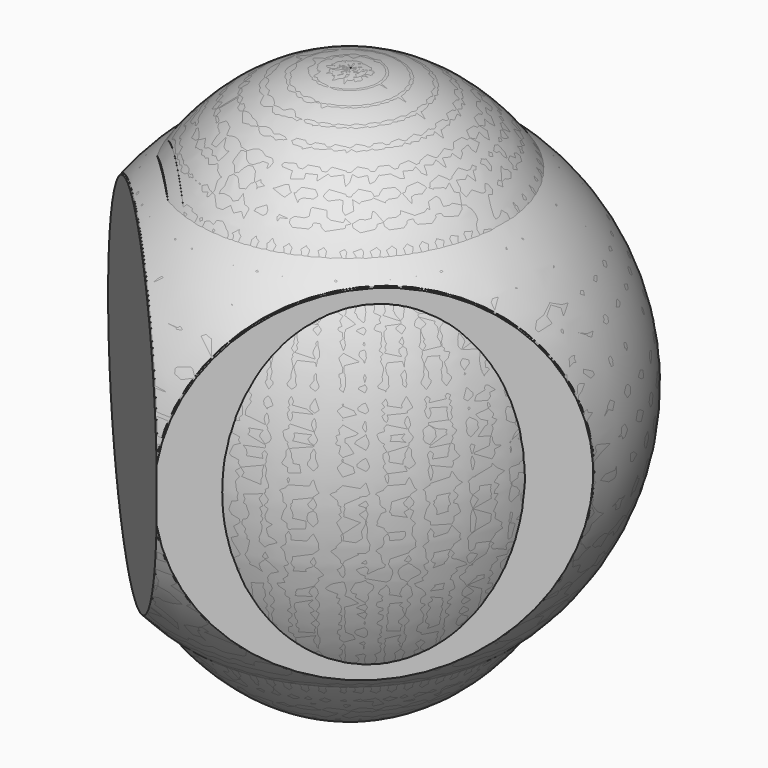
from build123d import *

# Parameters (mm, degrees)
F3_DEPTH       = 20.0010001
F3_DEPTH_BACK  = 25
F5_R           = 4
F6_DEPTH       = 8
F10_DEPTH      = 20.0010001
F10_DEPTH_BACK = 25
F13_R          = 4
F14_DEPTH      = 11.78
F18_DEPTH      = 20.0009988318
F18_DEPTH_BACK = 25
F20_R          = 4
F21_DEPTH      = 8
F25_DEPTH      = 20.0009988318
F25_DEPTH_BACK = 25
F28_R          = 4
F29_DEPTH      = 9.69
F33_R          = 1.486505693
F34_DEPTH      = 5


with BuildPart() as f1:
    # F0 (on Front) → F1 (revolve)
    with BuildSketch(Plane.XZ):
        with BuildLine():
            Line((0, 20), (0, -20))
            add(Edge.make_bspline(
                [(0, -20), (15, -20), (15, 0), (15, 20), (0, 20)],
                knots=[0, 0, 0, 1.5707963268, 1.5707963268, 3.1415926536, 3.1415926536, 3.1415926536], degree=2, weights=[1, 0.7071067812, 1, 0.7071067812, 1]))
        make_face()
    revolve(axis=Axis((0, 0, 1.515686512), (0, 0, -1)))

    # F2 (on Top) → F3 (cut, two sides)
    with BuildSketch(Plane.XY) as f3_sk:
        Polygon((1.0869333055, -18.0716644973), (1.0869333055, -15.0260711089), (-14.0562849119, 0), (1.0869333055, 14.9701479822), (1.0869333055, 17.4571201205), (-20.6206664443, 17.9764218628), (-19.673416391, -17.4401663244), align=None)
    extrude(amount=F3_DEPTH, mode=Mode.SUBTRACT)
    extrude(f3_sk.sketch, amount=-F3_DEPTH_BACK, mode=Mode.SUBTRACT)

    # F5 (on offset) → F6 (cut)
    with BuildSketch(Plane.XY.offset(-20.2)):
        Circle(F5_R)
    extrude(amount=F6_DEPTH, mode=Mode.SUBTRACT)


with BuildPart() as f8:
    # F7 (on Front) → F8 (revolve)
    with BuildSketch(Plane.XZ):
        with BuildLine():
            Line((0, 20), (0, -20))
            add(Edge.make_bspline(
                [(0, -20), (15, -20), (15, 0), (15, 20), (0, 20)],
                knots=[3.1415926536, 3.1415926536, 3.1415926536, 4.7123889804, 4.7123889804, 6.2831853072, 6.2831853072, 6.2831853072], degree=2, weights=[1, 0.7071067812, 1, 0.7071067812, 1]))
        make_face()
    revolve(axis=Axis((0, 0, 0), (0, 0, -1)))

    # F9 (on Top) → F10 (cut, two sides)
    with BuildSketch(Plane.XY) as f10_sk:
        Polygon((-19.6712000702, -17.4563237451), (2.0983788266, -17.0855390455), (-14.9871602189, 0), (3.7128583062, 18.7000185251), (-20.6184501235, 17.9602644421), align=None)
    extrude(amount=F10_DEPTH, mode=Mode.SUBTRACT)
    extrude(f10_sk.sketch, amount=-F10_DEPTH_BACK, mode=Mode.SUBTRACT)

    # F13 (on face) → F14 (cut)
    with BuildSketch(Plane(origin=(6.3216225389, 0, -23.5926165013), x_dir=(0.9659258263, 0, 0.2588190451), z_dir=(0.2588190451, 0, -0.9659258263))):
        with Locations((-1.1815404284, 0)):
            Circle(F13_R)
    extrude(amount=-F14_DEPTH, mode=Mode.SUBTRACT)


with BuildPart() as f16:
    # F15 (on Front) → F16 (revolve)
    with BuildSketch(Plane.XZ):
        with BuildLine():
            Line((0, 17.524996667), (0, -17.475003333))
            ThreePointArc((0, -17.475003333), (17.5, 0.024996667), (0, 17.524996667))
        make_face()
    revolve(axis=Axis((0, 0, 0.024996667), (0, 0, 1)))

    # F17 (on Top) → F18 (cut, two sides)
    with BuildSketch(Plane.XY) as f18_sk:
        Polygon((19.9882806891, 2.7019725794), (0, -17.2863081098), (-21.6209556736, 4.3346475638), (-21.6209556736, -23.6485283822), (21.9593252987, -24.4044363499), align=None)
    extrude(amount=-F18_DEPTH, mode=Mode.SUBTRACT)
    extrude(f18_sk.sketch, amount=F18_DEPTH_BACK, mode=Mode.SUBTRACT)

    # F20 (on offset) → F21 (cut)
    with BuildSketch(Plane.XY.offset(-17.5)):
        with Locations((0.0065488625, 0.0003273475)):
            Circle(F20_R)
    extrude(amount=F21_DEPTH, mode=Mode.SUBTRACT)


with BuildPart() as f23:
    # F22 (on Front) → F23 (revolve)
    with BuildSketch(Plane.XZ):
        with BuildLine():
            Line((0, 17.5), (0, -17.5))
            ThreePointArc((0, -17.5), (17.5, 0), (0, 17.5))
        make_face()
    revolve(axis=Axis((0, 0, 0), (0, 0, 1)))

    # F24 (on Top) → F25 (cut, two sides)
    with BuildSketch(Plane.XY) as f25_sk:
        Polygon((22.5941926348, 5.1994469124), (0, -17.3947457224), (-21.6209556736, 4.2262099512), (-21.6209556736, -25.0878847816), (21.6209556736, -25.8428923846), align=None)
    extrude(amount=-F25_DEPTH, mode=Mode.SUBTRACT)
    extrude(f25_sk.sketch, amount=F25_DEPTH_BACK, mode=Mode.SUBTRACT)

    # F28 (on face) → F29 (cut)
    with BuildSketch(Plane(origin=(0, 5.3318575956, -19.8987634455), x_dir=(1, 0, 0), z_dir=(0, 0.2588190451, -0.9659258263))):
        with Locations((0, 0.5199451661)):
            Circle(F28_R)
    extrude(amount=-F29_DEPTH, mode=Mode.SUBTRACT)


with BuildPart() as f31:
    # F30 (on Front) → F31 (revolve)
    with BuildSketch(Plane.XZ):
        with BuildLine():
            Line((0, 0), (6, 0))
            ThreePointArc((6, 0), (4.2426406871, 4.2426406871), (0, 6))
            Line((0, 6), (0, 0))
        make_face()
    revolve(axis=Axis((3, 0, 0), (1, 0, 0)))

    # F33 (on offset) → F34 (cut)
    with BuildSketch(Plane.XY.offset(6)):
        with Locations((2.5, 0)):
            Circle(F33_R)
    extrude(amount=-F34_DEPTH, mode=Mode.SUBTRACT)


solid = Compound([f1.part, f8.part, f16.part, f23.part, f31.part])
